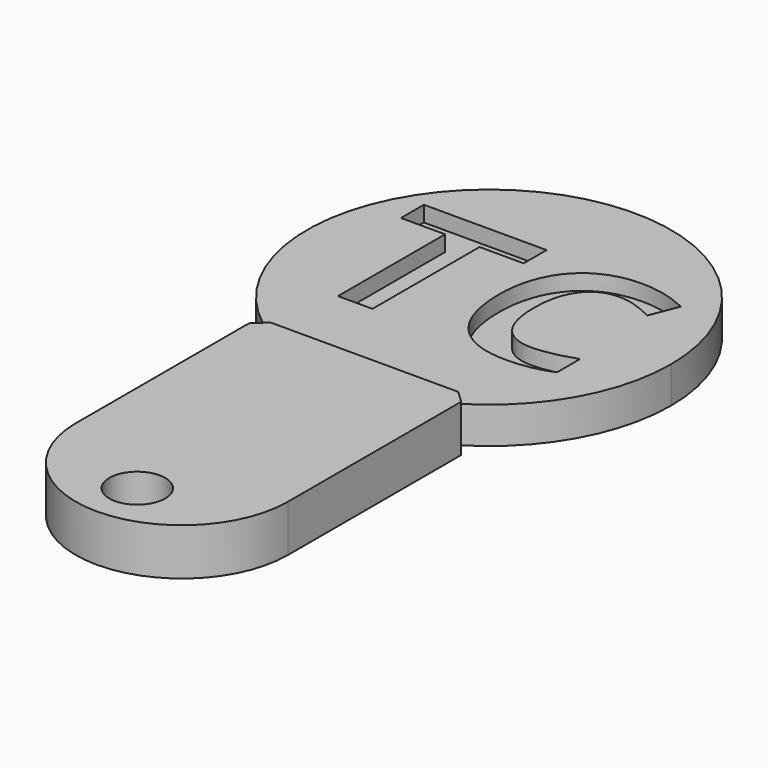
from build123d import *

# Parameters (mm, degrees)
F1_DEPTH     = 2.33
F2_R         = 1.7857519064
F3_DEPTH     = 3
F4_TEXT_SIZE = 14.5464076221
F5_DEPTH     = 1


# Not quite as in the source:
# - Text() gives the source's letters only with a copy of the font that has no kerning and outlines rounded to 1/6400 em; it was checked with that copy


with BuildPart() as f1:
    # F0 (on Top) → F1 (new body)
    with BuildSketch(Plane.XY):
        with BuildLine():
            ThreePointArc((6, -9.9569385355), (10.1215271822, -5.7179815057), (11.625, 0))
            ThreePointArc((11.625, 0), (-5.7179815057, 10.1215271822), (-6, -9.9569385355))
            Line((-6, -9.9569385355), (6, -9.9569385355))
        make_face()
    extrude(amount=F1_DEPTH)

    # F2 (on Top) → F3 (join)
    with BuildSketch(Plane.XY):
        with BuildLine():
            Line((6, -9.9569385355), (-6, -9.9569385355))
            Line((-6, -9.9569385355), (-6.7806313746, -10.6990638152))
            Line((-6.7806313746, -10.6990638152), (-6.7806313746, -24.5322883129))
            ThreePointArc((-6.7806313746, -24.5322883129), (0, -31.3129196875), (6.7806313746, -24.5322883129))
            Line((6.7806313746, -24.5322883129), (6.7806313746, -10.6990638152))
            Line((6.7806313746, -10.6990638152), (6, -9.9569385355))
        make_face()
        with Locations((0, -28.090134263)):
            Circle(F2_R, mode=Mode.SUBTRACT)
    extrude(amount=F3_DEPTH)

    # F4 (on face) → F5 (cut)
    with BuildSketch(Plane.XY.offset(2.33)):
        with Locations((-9.0619573733, -4.6232014215)):
            Text('TC', F4_TEXT_SIZE, font='Open Sans', font_style=FontStyle.BOLD, text_align=(TextAlign.LEFT, TextAlign.BOTTOM))
    extrude(amount=-F5_DEPTH, mode=Mode.SUBTRACT)


solid = f1.part
